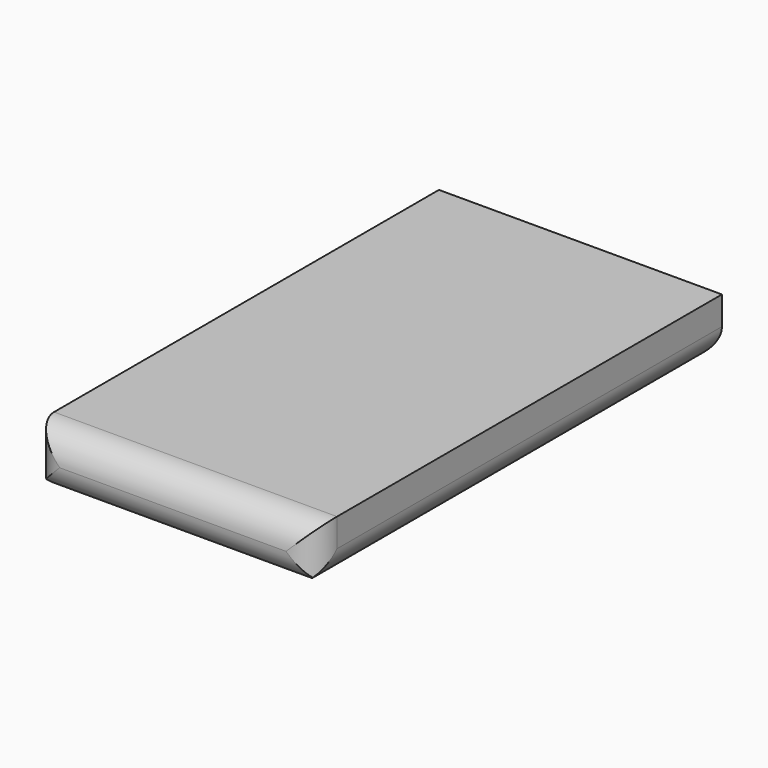
from build123d import *

# Parameters (mm, degrees)
F0_W        = 250
F0_H        = 450
F1_DEPTH    = 50
F2_R        = 24.99999
F3_T1_DEPTH = 550.00001
F3_T3_DEPTH = 375


# Not quite as in the source:
# - a fillet or chamfer that OpenCascade refuses, or shapes differently, is made with other operations: its cross-section is extruded or revolved along the edge and cut away or added
# - a fillet or chamfer is up to 0.001 mm smaller than in the source, because OpenCascade refuses the exact size


with BuildPart() as f1:
    # F0 (on Top) → F1 (new body)
    with BuildSketch(Plane.XY):
        Rectangle(F0_W, F0_H)
    extrude(amount=F1_DEPTH)

    # F2 (radius 25 in the source; OpenCascade refuses exactly that, so slightly less here)
    f2_edges = [f1.edges().sort_by_distance(p)[0] for p in [
        (-125, -225, 25),
        (125, -225, 25),
        (0, -225, 0),
        (0, -225, 50),
    ]]
    fillet(f2_edges, radius=F2_R)

    # F3: fillet of radius 25 on 4 edges, made by hand

    # F3_s2 → F3_t1 (cut)
    with BuildSketch(Plane.XZ.offset(-287.5)):
        with BuildLine():
            ThreePointArc((-125, 25), (-117.6776695297, 7.3223304703), (-100, 0))
            Line((-100, 0), (-125, 0))
            Line((-125, 0), (-125, 25))
        make_face()
        with BuildLine():
            ThreePointArc((100, 0), (117.6776695297, 7.3223304703), (125, 25))
            Line((125, 25), (125, 0))
            Line((125, 0), (100, 0))
        make_face()
    extrude(amount=F3_T1_DEPTH, mode=Mode.SUBTRACT)

    # F3_s4 → F3_t3 (cut)
    with BuildSketch(Plane.YZ.offset(-187.5)):
        with BuildLine():
            ThreePointArc((200, 0), (217.6776695297, 7.3223304703), (225, 25))
            Line((225, 25), (225, 0))
            Line((225, 0), (200, 0))
        make_face()
    extrude(amount=F3_T3_DEPTH, mode=Mode.SUBTRACT)


solid = f1.part
